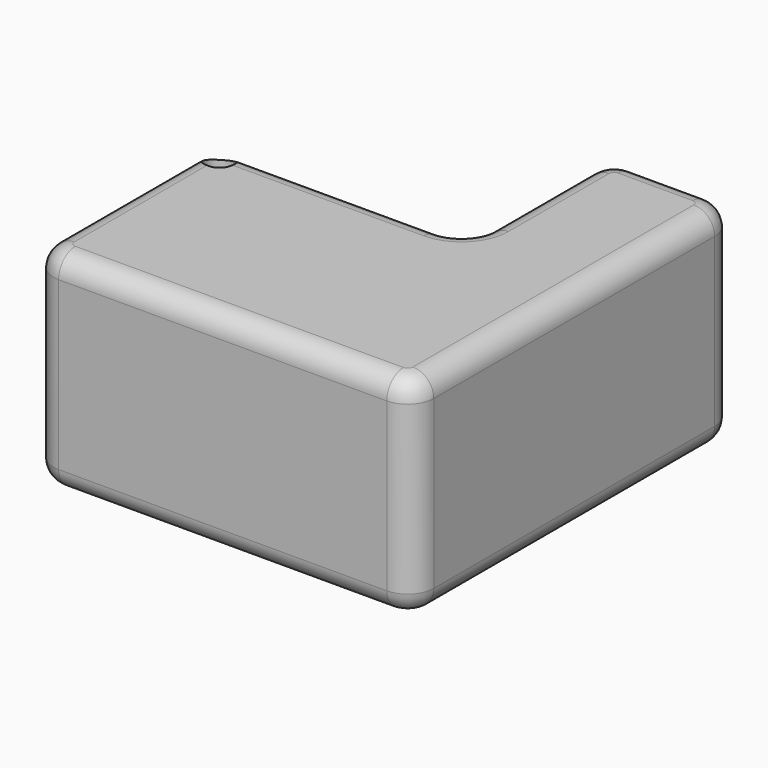
from build123d import *

# Parameters (mm, degrees)
F0_R         = 3.3955807327
F1_DEPTH     = 50.8
F2_T1_DEPTH  = 79.7933701754
F2_T3_DEPTH  = 85.3559065938
F2_T5_DEPTH  = 18.0880006731
F2_T7_DEPTH  = 30.5066917419
F2_T9_DEPTH  = 49.0053695023
F2_T11_DEPTH = 42.1492148519
F2_T14_ANGLE = 90
F2_T16_ANGLE = 90
F2_T18_ANGLE = 90
F2_T20_ANGLE = 90
F2_T22_ANGLE = 90
F2_T24_ANGLE = 90
F2_T26_ANGLE = 90
F2_T28_ANGLE = 90
F2_T30_ANGLE = 90
F2_T32_ANGLE = 90
F2_T34_ANGLE = 90
F2_T36_ANGLE = 90


# Not quite as in the source:
# - a fillet or chamfer that OpenCascade refuses, or shapes differently, is made with other operations: its cross-section is extruded or revolved along the edge and cut away or added


with BuildPart() as f1:
    # F0 (on Top) → F1 (new body)
    with BuildSketch(Plane.XY):
        with BuildLine():
            Line((12.9895242095, 20.2450528741), (-36.0158452928, 20.2450528741))
            ThreePointArc((-36.0158452928, 20.2450528741), (-40.5059733533, 18.3851809346), (-42.3658452928, 13.8950528741))
            Line((-42.3658452928, 13.8950528741), (-42.3658452928, -28.2541619778))
            ThreePointArc((-42.3658452928, -28.2541619778), (-40.5059733533, -32.7442900383), (-36.0158452928, -34.6041619778))
            Line((-36.0158452928, -34.6041619778), (43.7775248826, -34.6041619778))
            ThreePointArc((43.7775248826, -34.6041619778), (48.2676529431, -32.7442900383), (50.1275248826, -28.2541619778))
            Line((50.1275248826, -28.2541619778), (50.1275248826, 20.2450528741))
            Line((50.1275248826, 20.2450528741), (50.1275248826, 57.101744616))
            ThreePointArc((50.1275248826, 57.101744616), (48.2676529431, 61.5918726766), (43.7775248826, 63.451744616))
            Line((43.7775248826, 63.451744616), (25.6895242095, 63.451744616))
            ThreePointArc((25.6895242095, 63.451744616), (21.199396149, 61.5918726766), (19.3395242095, 57.101744616))
            Line((19.3395242095, 57.101744616), (19.3395242095, 26.5950528741))
            ThreePointArc((19.3395242095, 26.5950528741), (17.47965227, 22.1049248136), (12.9895242095, 20.2450528741))
        make_face()
        with Locations((-36.93266958, 15.458682552)):
            Circle(F0_R, mode=Mode.SUBTRACT)
    extrude(amount=F1_DEPTH)

    # F2: fillet of radius 5.08 on 2 edges, made by hand

    # F2_s2 → F2_t1 (cut)
    with BuildSketch(Plane.YZ.offset(-36.0158452928)):
        with BuildLine():
            ThreePointArc((-29.5241619778, 50.8), (-33.1162644262, 49.3121024484), (-34.6041619778, 45.72))
            Line((-34.6041619778, 45.72), (-34.6041619778, 50.8))
            Line((-34.6041619778, 50.8), (-29.5241619778, 50.8))
        make_face()
        with BuildLine():
            ThreePointArc((-34.6041619778, 5.08), (-33.1162644262, 1.4878975516), (-29.5241619778, 0))
            Line((-29.5241619778, 0), (-34.6041619778, 0))
            Line((-34.6041619778, 0), (-34.6041619778, 5.08))
        make_face()
    extrude(amount=F2_T1_DEPTH, mode=Mode.SUBTRACT)

    # F2_s4 → F2_t3 (cut)
    with BuildSketch(Plane.XZ.offset(-57.101744616)):
        with BuildLine():
            ThreePointArc((50.1275248826, 5.08), (48.639627331, 1.4878975516), (45.0475248826, 0))
            Line((45.0475248826, 0), (50.1275248826, 0))
            Line((50.1275248826, 0), (50.1275248826, 5.08))
        make_face()
        with BuildLine():
            ThreePointArc((45.0475248826, 50.8), (48.639627331, 49.3121024484), (50.1275248826, 45.72))
            Line((50.1275248826, 45.72), (50.1275248826, 50.8))
            Line((50.1275248826, 50.8), (45.0475248826, 50.8))
        make_face()
    extrude(amount=F2_T3_DEPTH, mode=Mode.SUBTRACT)

    # F2_s6 → F2_t5 (cut)
    with BuildSketch(Plane.YZ.offset(25.6895242095)):
        with BuildLine():
            ThreePointArc((63.451744616, 5.08), (61.9638470645, 1.4878975516), (58.371744616, 0))
            Line((58.371744616, 0), (63.451744616, 0))
            Line((63.451744616, 0), (63.451744616, 5.08))
        make_face()
        with BuildLine():
            ThreePointArc((58.371744616, 50.8), (61.9638470645, 49.3121024484), (63.451744616, 45.72))
            Line((63.451744616, 45.72), (63.451744616, 50.8))
            Line((63.451744616, 50.8), (58.371744616, 50.8))
        make_face()
    extrude(amount=F2_T5_DEPTH, mode=Mode.SUBTRACT)

    # F2_s8 → F2_t7 (cut)
    with BuildSketch(Plane.XZ.offset(-57.101744616)):
        with BuildLine():
            ThreePointArc((24.4195242095, 0), (20.8274217611, 1.4878975516), (19.3395242095, 5.08))
            Line((19.3395242095, 5.08), (19.3395242095, 0))
            Line((19.3395242095, 0), (24.4195242095, 0))
        make_face()
        with BuildLine():
            ThreePointArc((24.4195242095, 50.8), (20.8274217611, 49.3121024484), (19.3395242095, 45.72))
            Line((19.3395242095, 45.72), (19.3395242095, 50.8))
            Line((19.3395242095, 50.8), (24.4195242095, 50.8))
        make_face()
    extrude(amount=F2_T7_DEPTH, mode=Mode.SUBTRACT)

    # F2_s10 → F2_t9 (cut)
    with BuildSketch(Plane.YZ.offset(-36.0158452928)):
        with BuildLine():
            ThreePointArc((15.1650528741, 0), (18.7571553225, 1.4878975516), (20.2450528741, 5.08))
            Line((20.2450528741, 5.08), (20.2450528741, 0))
            Line((20.2450528741, 0), (15.1650528741, 0))
        make_face()
        with BuildLine():
            ThreePointArc((15.1650528741, 50.8), (18.7571553225, 49.3121024484), (20.2450528741, 45.72))
            Line((20.2450528741, 45.72), (20.2450528741, 50.8))
            Line((20.2450528741, 50.8), (15.1650528741, 50.8))
        make_face()
    extrude(amount=F2_T9_DEPTH, mode=Mode.SUBTRACT)

    # F2_s12 → F2_t11 (cut)
    with BuildSketch(Plane.XZ.offset(-13.8950528741)):
        with BuildLine():
            ThreePointArc((-42.3658452928, 5.08), (-40.8779477412, 1.4878975516), (-37.2858452928, 0))
            Line((-37.2858452928, 0), (-42.3658452928, 0))
            Line((-42.3658452928, 0), (-42.3658452928, 5.08))
        make_face()
        with BuildLine():
            ThreePointArc((-37.2858452928, 50.8), (-40.8779477412, 49.3121024484), (-42.3658452928, 45.72))
            Line((-42.3658452928, 45.72), (-42.3658452928, 50.8))
            Line((-42.3658452928, 50.8), (-37.2858452928, 50.8))
        make_face()
    extrude(amount=F2_T11_DEPTH, mode=Mode.SUBTRACT)

    # F2_s13 → F2_t14 (revolve, cut)
    with BuildSketch(Plane.XZ.offset(28.2541619778)):
        with BuildLine():
            ThreePointArc((-42.3658452928, 5.08), (-40.8779477412, 1.4878975516), (-37.2858452928, 0))
            Line((-37.2858452928, 0), (-42.3658452928, 0))
            Line((-42.3658452928, 0), (-42.3658452928, 5.08))
        make_face()
    revolve(axis=Axis((-36.0158452928, -28.2541619778, 0), (0, 0, 1)), revolution_arc=F2_T14_ANGLE, mode=Mode.SUBTRACT)

    # F2_s15 → F2_t16 (revolve, cut)
    with BuildSketch(Plane.YZ.offset(43.7775248826)):
        with BuildLine():
            ThreePointArc((-34.6041619778, 5.08), (-33.1162644262, 1.4878975516), (-29.5241619778, 0))
            Line((-29.5241619778, 0), (-34.6041619778, 0))
            Line((-34.6041619778, 0), (-34.6041619778, 5.08))
        make_face()
    revolve(axis=Axis((43.7775248826, -28.2541619778, 0), (0, 0, 1)), revolution_arc=F2_T16_ANGLE, mode=Mode.SUBTRACT)

    # F2_s17 → F2_t18 (revolve, cut)
    with BuildSketch(Plane.XZ.offset(-57.101744616)):
        with BuildLine():
            ThreePointArc((50.1275248826, 5.08), (48.639627331, 1.4878975516), (45.0475248826, 0))
            Line((45.0475248826, 0), (50.1275248826, 0))
            Line((50.1275248826, 0), (50.1275248826, 5.08))
        make_face()
    revolve(axis=Axis((43.7775248826, 57.101744616, 0), (0, 0, 1)), revolution_arc=F2_T18_ANGLE, mode=Mode.SUBTRACT)

    # F2_s19 → F2_t20 (revolve, cut)
    with BuildSketch(Plane.YZ.offset(25.6895242095)):
        with BuildLine():
            ThreePointArc((63.451744616, 5.08), (61.9638470645, 1.4878975516), (58.371744616, 0))
            Line((58.371744616, 0), (63.451744616, 0))
            Line((63.451744616, 0), (63.451744616, 5.08))
        make_face()
    revolve(axis=Axis((25.6895242095, 57.101744616, 0), (0, 0, 1)), revolution_arc=F2_T20_ANGLE, mode=Mode.SUBTRACT)

    # F2_s21 → F2_t22 (revolve, cut)
    with BuildSketch(Plane.XZ.offset(-26.5950528741)):
        with BuildLine():
            ThreePointArc((19.3395242095, 5.08), (20.8274217611, 1.4878975516), (24.4195242095, 0))
            Line((24.4195242095, 0), (19.3395242095, 0))
            Line((19.3395242095, 0), (19.3395242095, 5.08))
        make_face()
    revolve(axis=Axis((12.9895242095, 26.5950528741, 0), (0, 0, -1)), revolution_arc=F2_T22_ANGLE, mode=Mode.SUBTRACT)

    # F2_s23 → F2_t24 (revolve, cut)
    with BuildSketch(Plane.YZ.offset(-36.0158452928)):
        with BuildLine():
            ThreePointArc((20.2450528741, 5.08), (18.7571553225, 1.4878975516), (15.1650528741, 0))
            Line((15.1650528741, 0), (20.2450528741, 0))
            Line((20.2450528741, 0), (20.2450528741, 5.08))
        make_face()
    revolve(axis=Axis((-36.0158452928, 13.8950528741, 0), (0, 0, 1)), revolution_arc=F2_T24_ANGLE, mode=Mode.SUBTRACT)

    # F2_s25 → F2_t26 (revolve, cut)
    with BuildSketch(Plane.XZ.offset(28.2541619778)):
        with BuildLine():
            ThreePointArc((-37.2858452928, 50.8), (-40.8779477412, 49.3121024484), (-42.3658452928, 45.72))
            Line((-42.3658452928, 45.72), (-42.3658452928, 50.8))
            Line((-42.3658452928, 50.8), (-37.2858452928, 50.8))
        make_face()
    revolve(axis=Axis((-36.0158452928, -28.2541619778, 50.8), (0, 0, 1)), revolution_arc=F2_T26_ANGLE, mode=Mode.SUBTRACT)

    # F2_s27 → F2_t28 (revolve, cut)
    with BuildSketch(Plane.YZ.offset(43.7775248826)):
        with BuildLine():
            ThreePointArc((-29.5241619778, 50.8), (-33.1162644262, 49.3121024484), (-34.6041619778, 45.72))
            Line((-34.6041619778, 45.72), (-34.6041619778, 50.8))
            Line((-34.6041619778, 50.8), (-29.5241619778, 50.8))
        make_face()
    revolve(axis=Axis((43.7775248826, -28.2541619778, 50.8), (0, 0, 1)), revolution_arc=F2_T28_ANGLE, mode=Mode.SUBTRACT)

    # F2_s29 → F2_t30 (revolve, cut)
    with BuildSketch(Plane.XZ.offset(-57.101744616)):
        with BuildLine():
            ThreePointArc((45.0475248826, 50.8), (48.639627331, 49.3121024484), (50.1275248826, 45.72))
            Line((50.1275248826, 45.72), (50.1275248826, 50.8))
            Line((50.1275248826, 50.8), (45.0475248826, 50.8))
        make_face()
    revolve(axis=Axis((43.7775248826, 57.101744616, 50.8), (0, 0, 1)), revolution_arc=F2_T30_ANGLE, mode=Mode.SUBTRACT)

    # F2_s31 → F2_t32 (revolve, cut)
    with BuildSketch(Plane.YZ.offset(25.6895242095)):
        with BuildLine():
            ThreePointArc((58.371744616, 50.8), (61.9638470645, 49.3121024484), (63.451744616, 45.72))
            Line((63.451744616, 45.72), (63.451744616, 50.8))
            Line((63.451744616, 50.8), (58.371744616, 50.8))
        make_face()
    revolve(axis=Axis((25.6895242095, 57.101744616, 50.8), (0, 0, 1)), revolution_arc=F2_T32_ANGLE, mode=Mode.SUBTRACT)

    # F2_s33 → F2_t34 (revolve, cut)
    with BuildSketch(Plane.XZ.offset(-26.5950528741)):
        with BuildLine():
            ThreePointArc((19.3395242095, 45.72), (20.8274217611, 49.3121024484), (24.4195242095, 50.8))
            Line((24.4195242095, 50.8), (19.3395242095, 50.8))
            Line((19.3395242095, 50.8), (19.3395242095, 45.72))
        make_face()
    revolve(axis=Axis((12.9895242095, 26.5950528741, 50.8), (0, 0, -1)), revolution_arc=F2_T34_ANGLE, mode=Mode.SUBTRACT)

    # F2_s35 → F2_t36 (revolve, cut)
    with BuildSketch(Plane.YZ.offset(-36.0158452928)):
        with BuildLine():
            ThreePointArc((15.1650528741, 50.8), (18.7571553225, 49.3121024484), (20.2450528741, 45.72))
            Line((20.2450528741, 45.72), (20.2450528741, 50.8))
            Line((20.2450528741, 50.8), (15.1650528741, 50.8))
        make_face()
    revolve(axis=Axis((-36.0158452928, 13.8950528741, 50.8), (0, 0, 1)), revolution_arc=F2_T36_ANGLE, mode=Mode.SUBTRACT)


solid = f1.part
